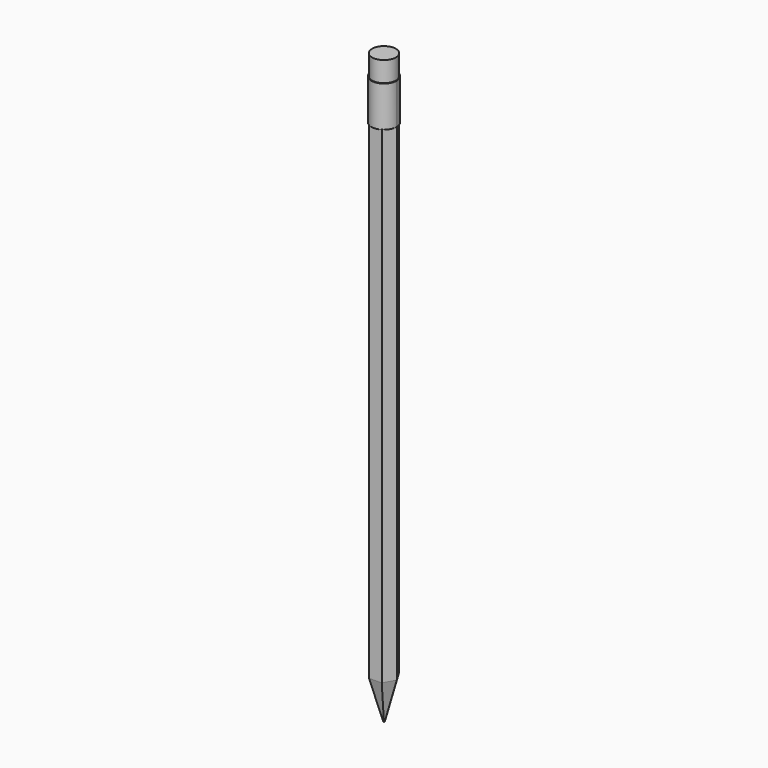
from build123d import *

# Parameters (mm, degrees)
F1_DEPTH = 152.4
F3_DEPTH = 12.7
F4_R     = 3.7116770234
F5_DEPTH = 6.35
F7_R     = 0.2026181046


with BuildPart() as f1:
    # F0 (on Top) → F1 (new body)
    with BuildSketch(Plane.XY):
        Polygon((22.5227356887, 13.1351892635), (20.5084380472, 16.5440003483), (16.5491722304, 16.5039729623), (14.604204055, 13.0551344916), (16.6185016965, 9.6463234069), (20.5777675134, 9.6863507928), align=None)
    extrude(amount=F1_DEPTH)

    # F1_face (on face) + F1_face1 (on face) + F2 (on face) → F3 (join)
    with BuildSketch(Plane(origin=(18.5634698719, 13.0951618776, 152.4), x_dir=(1, 0, 0), z_dir=(0, 0, 1))):
        Polygon((3.9592658168, 0.0400273859), (1.9449681753, 3.4488384707), (-2.0142976415, 3.4088110847), (-3.9592658168, -0.0400273859), (-1.9449681753, -3.4488384707), (2.0142976415, -3.4088110847), align=None)
    with BuildSketch(Plane(origin=(18.5634698719, 13.0951618776, 0), x_dir=(1, 0, 0), z_dir=(0, 0, -1))):
        Polygon((1.9449681753, -3.4488384707), (3.9592658168, -0.0400273859), (2.0142976415, 3.4088110847), (-1.9449681753, 3.4488384707), (-3.9592658168, 0.0400273859), (-2.0142976415, -3.4088110847), align=None)
    with BuildSketch(Plane.XY.offset(152.4)):
        with BuildLine():
            ThreePointArc((14.604204055, 13.0551344916), (18.5753456023, 9.1190642761), (22.5231408121, 13.0785499639))
            ThreePointArc((22.5231408121, 13.0785499639), (22.5230395299, 13.1068703381), (22.5227356887, 13.1351892635))
            Line((22.5227356887, 13.1351892635), (20.5777675134, 9.6863507928))
            Line((20.5777675134, 9.6863507928), (16.6185016965, 9.6463234069))
            Line((16.6185016965, 9.6463234069), (14.604204055, 13.0551344916))
        make_face()
        with BuildLine():
            Line((20.5230763012, 16.5192279208), (22.5227356887, 13.1351892635))
            ThreePointArc((22.5227356887, 13.1351892635), (21.9724789039, 15.0928653351), (20.5230763012, 16.5192279208))
        make_face()
        with BuildLine():
            Line((20.5777675134, 9.6863507928), (22.5227356887, 13.1351892635))
            Line((22.5227356887, 13.1351892635), (20.5230763012, 16.5192279208))
            ThreePointArc((20.5230763012, 16.5192279208), (20.501303397, 16.5315365084), (20.4794531772, 16.543707317))
            Line((20.4794531772, 16.543707317), (16.5781571004, 16.5042659936))
            ThreePointArc((16.5781571004, 16.5042659936), (16.5565574105, 16.491655915), (16.5350378058, 16.4789096488))
            Line((16.5350378058, 16.4789096488), (14.604204055, 13.0551344916))
            Line((14.604204055, 13.0551344916), (16.6185016965, 9.6463234069))
            Line((16.6185016965, 9.6463234069), (20.5777675134, 9.6863507928))
        make_face()
        with BuildLine():
            ThreePointArc((16.5350378058, 16.4789096488), (15.1147689879, 15.0235352587), (14.604204055, 13.0551344916))
            Line((14.604204055, 13.0551344916), (16.5350378058, 16.4789096488))
        make_face()
        with BuildLine():
            Line((16.5781571004, 16.5042659936), (20.4794531772, 16.543707317))
            ThreePointArc((20.4794531772, 16.543707317), (18.5236100767, 17.0378506299), (16.5781571004, 16.5042659936))
        make_face()
    extrude(amount=F3_DEPTH, dir=(0, 0, 1))

    # F4 (on face) → F5 (join)
    with BuildSketch(Plane.XY.offset(165.1)):
        with Locations((18.563637815, 13.0785499639)):
            Circle(F4_R)
    extrude(amount=F5_DEPTH)

    # F1_face1 (on face) → F8 section 0
    with BuildSketch(Plane(origin=(18.5634698719, 13.0951618776, 0), x_dir=(1, 0, 0), z_dir=(0, 0, -1))):
        Polygon((1.9449681753, -3.4488384707), (3.9592658168, -0.0400273859), (2.0142976415, 3.4088110847), (-1.9449681753, 3.4488384707), (-3.9592658168, 0.0400273859), (-2.0142976415, -3.4088110847), align=None)
    # F7 (on offset) → F8 section 1
    with BuildSketch(Plane(origin=(0, 0, -12.7), x_dir=(1, 0, 0), z_dir=(0, 0, -1))):
        with Locations((18.5634698719, -13.0951618776)):
            Circle(F7_R)
    loft()


solid = f1.part
